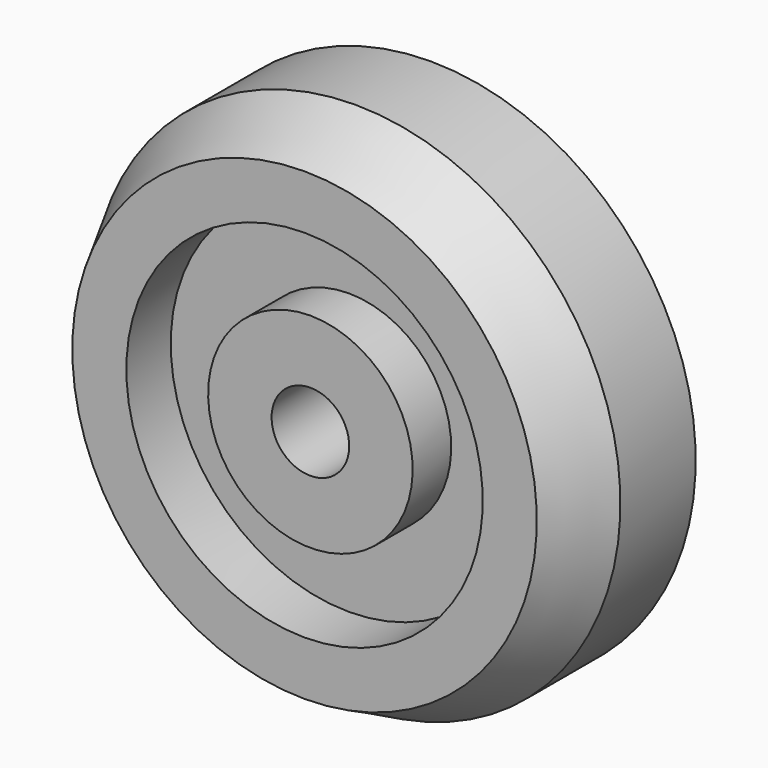
from build123d import *


# Not quite as in the source:
# - a feature of the source that left no trace in its solid (it failed there, or was rolled back) is left out


with BuildPart() as f1:
    # F0 (on Right) → F1 (revolve)
    with BuildSketch(Plane.YZ):
        Polygon((34.94284302, 67.0327916741), (18.8470929861, 58.7586164474), (18.8470929861, 45.085221529), (32.8900367022, 45.085221529), (32.8900367022, 25.8685648441), (20.6948518753, 25.8685648441), (20.6948518753, 9.8165124655), (54.5071139932, 9.8165124655), (54.5071139932, 26.4276862144), (45.0941175222, 26.4276862144), (45.0941175222, 46.3611036539), (58.752194047, 46.3611036539), (58.752194047, 67.0327916741), align=None)
    revolve(axis=Axis((0, 36.2159982324, 0), (0, 1, 0)))


solid = f1.part
